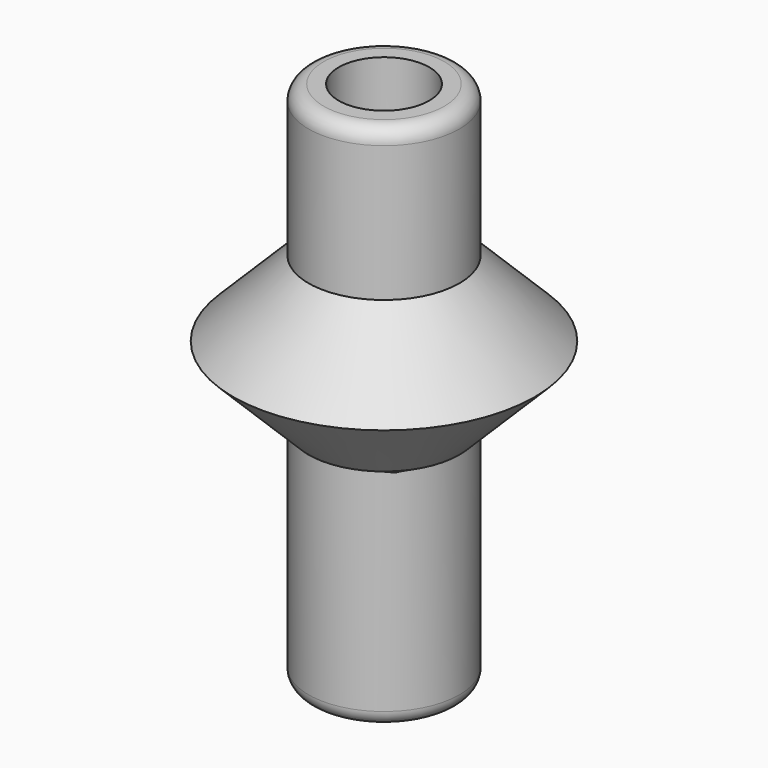
from build123d import *

# Parameters (mm, degrees)
F0_R         = 12.7
F1_DEPTH     = 38.1
F2_R         = 25.4
F2_R_2       = 12.7
F3_DEPTH     = 12.7
F4_R         = 2.54
F5_T1_DEPTH  = 10.7763073453
F5_T3_DEPTH  = 10.7763073453
F5_T9_DEPTH  = 23.4763073453
F5_S10_R     = 12.7
F5_T11_DEPTH = 14
F5_T15_DEPTH = 23.4763073453
F5_S16_R     = 12.7
F5_T17_DEPTH = 14
F5_T24_DEPTH = 23.4763073453
F5_S25_R     = 12.7
F5_T26_DEPTH = 14
F5_T30_DEPTH = 23.4763073453
F5_S31_R     = 12.7
F5_T32_DEPTH = 14
F5_T39_DEPTH = 23.4763073453
F5_S40_R     = 12.7
F5_T41_DEPTH = 14
F5_T45_DEPTH = 23.4763073453
F5_S46_R     = 12.7
F5_T47_DEPTH = 14
F5_T54_DEPTH = 23.4763073453
F5_S55_R     = 12.7
F5_T56_DEPTH = 14
F5_T60_DEPTH = 23.4763073453
F5_S61_R     = 12.7
F5_T62_DEPTH = 14
F8_R         = 12.7
F8_R_2       = 7.62
F9_DEPTH     = 25.4
F10_R        = 2.54
F11_DEPTH    = 25.4
F12_SIZE     = 12.69999
F13_R        = 2.54
F14_DEPTH    = 152.4


# Not quite as in the source:
# - a fillet or chamfer that OpenCascade refuses, or shapes differently, is made with other operations: its cross-section is extruded or revolved along the edge and cut away or added
# - a fillet or chamfer is up to 0.001 mm smaller than in the source, because OpenCascade refuses the exact size


with BuildPart() as f1:
    # F0 (on Top) → F1 (new body)
    with BuildSketch(Plane.XY):
        Circle(F0_R)
        with BuildLine():
            ThreePointArc((5.3881536726, 5.3881536726), (7.0399620377, 2.9160477546), (7.62, 0))
            ThreePointArc((7.62, 0), (7.0399620377, -2.9160477546), (5.3881536726, -5.3881536726))
            ThreePointArc((5.3881536726, -5.3881536726), (0, -7.62), (-5.3881536726, -5.3881536726))
            ThreePointArc((-5.3881536726, -5.3881536726), (-7.62, 0), (-5.3881536726, 5.3881536726))
            ThreePointArc((-5.3881536726, 5.3881536726), (0, 7.62), (5.3881536726, 5.3881536726))
        make_face(mode=Mode.SUBTRACT)
        with BuildLine():
            ThreePointArc((-5.3881536726, -5.3881536726), (0, -7.62), (5.3881536726, -5.3881536726))
            Line((5.3881536726, -5.3881536726), (-5.3881536726, -5.3881536726))
        make_face()
        with BuildLine():
            Line((-5.3881536726, -5.3881536726), (-5.3881536726, 5.3881536726))
            ThreePointArc((-5.3881536726, 5.3881536726), (-7.62, 0), (-5.3881536726, -5.3881536726))
        make_face()
        with BuildLine():
            ThreePointArc((5.3881536726, -5.3881536726), (7.0399620377, -2.9160477546), (7.62, 0))
            ThreePointArc((7.62, 0), (7.0399620377, 2.9160477546), (5.3881536726, 5.3881536726))
            Line((5.3881536726, 5.3881536726), (5.3881536726, -5.3881536726))
        make_face()
        with BuildLine():
            Line((-5.3881536726, 5.3881536726), (5.3881536726, 5.3881536726))
            ThreePointArc((5.3881536726, 5.3881536726), (0, 7.62), (-5.3881536726, 5.3881536726))
        make_face()
    extrude(amount=F1_DEPTH)

    # F4
    f4_edges = [f1.edges().sort_by_distance(p)[0] for p in [
        (-12.7, 0, 0),
    ]]
    fillet(f4_edges, radius=F4_R)

    # F5: fillet of radius 5.08 on 4 edges, made by hand

    # F5_s2 → F5_t1 (cut)
    with BuildSketch(Plane.XZ.offset(-5.3881536726)):
        with BuildLine():
            ThreePointArc((10.4681536726, 38.1), (6.8760512242, 36.6121024484), (5.3881536726, 33.02))
            Line((5.3881536726, 33.02), (5.3881536726, 38.1))
            Line((5.3881536726, 38.1), (10.4681536726, 38.1))
        make_face()
        with BuildLine():
            ThreePointArc((-10.4681536726, 38.1), (-6.8760512242, 36.6121024484), (-5.3881536726, 33.02))
            Line((-5.3881536726, 33.02), (-5.3881536726, 38.1))
            Line((-5.3881536726, 38.1), (-10.4681536726, 38.1))
        make_face()
    extrude(amount=F5_T1_DEPTH, mode=Mode.SUBTRACT)

    # F5_s4 → F5_t3 (cut)
    with BuildSketch(Plane.YZ.offset(-5.3881536726)):
        with BuildLine():
            ThreePointArc((-10.4681536726, 38.1), (-6.8760512242, 36.6121024484), (-5.3881536726, 33.02))
            Line((-5.3881536726, 33.02), (-5.3881536726, 38.1))
            Line((-5.3881536726, 38.1), (-10.4681536726, 38.1))
        make_face()
        with BuildLine():
            ThreePointArc((10.4681536726, 38.1), (6.8760512242, 36.6121024484), (5.3881536726, 33.02))
            Line((5.3881536726, 33.02), (5.3881536726, 38.1))
            Line((5.3881536726, 38.1), (10.4681536726, 38.1))
        make_face()
    extrude(amount=F5_T3_DEPTH, mode=Mode.SUBTRACT)


with BuildPart() as f3:
    # F2 (on face) → F3 (new body)
    with BuildSketch(Plane.XY.offset(38.1)):
        Circle(F2_R)
        Circle(F2_R_2, mode=Mode.SUBTRACT)
    extrude(amount=F3_DEPTH)

    # F6: F3 across face


with BuildPart() as f5_tool7:
    # F5_s8 → F5_t9 (new body)
    with BuildSketch(Plane.YZ.offset(-5.3881536726)):
        with BuildLine():
            ThreePointArc((10.4681536726, 38.1), (6.8760512242, 36.6121024484), (5.3881536726, 33.02))
            Line((5.3881536726, 33.02), (5.3881536726, 38.1))
            Line((5.3881536726, 38.1), (10.4681536726, 38.1))
        make_face()
    extrude(amount=F5_T9_DEPTH)

    # F5_s10 → F5_t11 (intersect, symmetric)
    with BuildSketch(Plane.XY.offset(35.6)):
        Circle(F5_S10_R)
    extrude(amount=F5_T11_DEPTH, both=True, mode=Mode.INTERSECT)

    split(bisect_by=Plane.YZ.offset(5.3881536726), keep=Keep.TOP)


with BuildPart() as f5_tool13:
    # F5_s14 → F5_t15 (new body)
    with BuildSketch(Plane.XZ.offset(-18.0881536726)):
        with BuildLine():
            ThreePointArc((10.4681536726, 38.1), (6.8760512242, 36.6121024484), (5.3881536726, 33.02))
            Line((5.3881536726, 33.02), (5.3881536726, 38.1))
            Line((5.3881536726, 38.1), (10.4681536726, 38.1))
        make_face()
    extrude(amount=F5_T15_DEPTH)

    # F5_s16 → F5_t17 (intersect, symmetric)
    with BuildSketch(Plane.XY.offset(35.6)):
        Circle(F5_S16_R)
    extrude(amount=F5_T17_DEPTH, both=True, mode=Mode.INTERSECT)

    split(bisect_by=Plane.XZ.offset(-5.3881536726), keep=Keep.BOTTOM)


with BuildPart() as f5_tool7_1:
    add(f5_tool7.part)

    # F5_t19: intersect F5_tool13
    add(f5_tool13.part, mode=Mode.INTERSECT)


with BuildPart() as f1_1:
    add(f1.part)

    # F5_t5: cut F5_tool7
    add(f5_tool7_1.part, mode=Mode.SUBTRACT)


with BuildPart() as f5_tool22:
    # F5_s23 → F5_t24 (new body)
    with BuildSketch(Plane.YZ.offset(18.0881536726)):
        with BuildLine():
            ThreePointArc((-10.4681536726, 38.1), (-6.8760512242, 36.6121024484), (-5.3881536726, 33.02))
            Line((-5.3881536726, 33.02), (-5.3881536726, 38.1))
            Line((-5.3881536726, 38.1), (-10.4681536726, 38.1))
        make_face()
    extrude(amount=-F5_T24_DEPTH)

    # F5_s25 → F5_t26 (intersect, symmetric)
    with BuildSketch(Plane.XY.offset(35.6)):
        Circle(F5_S25_R)
    extrude(amount=F5_T26_DEPTH, both=True, mode=Mode.INTERSECT)

    split(bisect_by=Plane.YZ.offset(5.3881536726), keep=Keep.TOP)


with BuildPart() as f5_tool28:
    # F5_s29 → F5_t30 (new body)
    with BuildSketch(Plane.XZ.offset(-5.3881536726)):
        with BuildLine():
            ThreePointArc((10.4681536726, 38.1), (6.8760512242, 36.6121024484), (5.3881536726, 33.02))
            Line((5.3881536726, 33.02), (5.3881536726, 38.1))
            Line((5.3881536726, 38.1), (10.4681536726, 38.1))
        make_face()
    extrude(amount=F5_T30_DEPTH)

    # F5_s31 → F5_t32 (intersect, symmetric)
    with BuildSketch(Plane.XY.offset(35.6)):
        Circle(F5_S31_R)
    extrude(amount=F5_T32_DEPTH, both=True, mode=Mode.INTERSECT)

    split(bisect_by=Plane.XZ.offset(5.3881536726), keep=Keep.TOP)


with BuildPart() as f5_tool22_1:
    add(f5_tool22.part)

    # F5_t34: intersect F5_tool28
    add(f5_tool28.part, mode=Mode.INTERSECT)


with BuildPart() as f1_2:
    add(f1_1.part)

    # F5_t20: cut F5_tool22
    add(f5_tool22_1.part, mode=Mode.SUBTRACT)


with BuildPart() as f5_tool37:
    # F5_s38 → F5_t39 (new body)
    with BuildSketch(Plane.YZ.offset(5.3881536726)):
        with BuildLine():
            ThreePointArc((-10.4681536726, 38.1), (-6.8760512242, 36.6121024484), (-5.3881536726, 33.02))
            Line((-5.3881536726, 33.02), (-5.3881536726, 38.1))
            Line((-5.3881536726, 38.1), (-10.4681536726, 38.1))
        make_face()
    extrude(amount=-F5_T39_DEPTH)

    # F5_s40 → F5_t41 (intersect, symmetric)
    with BuildSketch(Plane.XY.offset(35.6)):
        Circle(F5_S40_R)
    extrude(amount=F5_T41_DEPTH, both=True, mode=Mode.INTERSECT)

    split(bisect_by=Plane.YZ.offset(-5.3881536726), keep=Keep.BOTTOM)


with BuildPart() as f5_tool43:
    # F5_s44 → F5_t45 (new body)
    with BuildSketch(Plane.XZ.offset(18.0881536726)):
        with BuildLine():
            ThreePointArc((-10.4681536726, 38.1), (-6.8760512242, 36.6121024484), (-5.3881536726, 33.02))
            Line((-5.3881536726, 33.02), (-5.3881536726, 38.1))
            Line((-5.3881536726, 38.1), (-10.4681536726, 38.1))
        make_face()
    extrude(amount=-F5_T45_DEPTH)

    # F5_s46 → F5_t47 (intersect, symmetric)
    with BuildSketch(Plane.XY.offset(35.6)):
        Circle(F5_S46_R)
    extrude(amount=F5_T47_DEPTH, both=True, mode=Mode.INTERSECT)

    split(bisect_by=Plane.XZ.offset(5.3881536726), keep=Keep.TOP)


with BuildPart() as f5_tool37_1:
    add(f5_tool37.part)

    # F5_t49: intersect F5_tool43
    add(f5_tool43.part, mode=Mode.INTERSECT)


with BuildPart() as f1_3:
    add(f1_2.part)

    # F5_t35: cut F5_tool37
    add(f5_tool37_1.part, mode=Mode.SUBTRACT)


with BuildPart() as f5_tool52:
    # F5_s53 → F5_t54 (new body)
    with BuildSketch(Plane.XZ.offset(5.3881536726)):
        with BuildLine():
            ThreePointArc((-10.4681536726, 38.1), (-6.8760512242, 36.6121024484), (-5.3881536726, 33.02))
            Line((-5.3881536726, 33.02), (-5.3881536726, 38.1))
            Line((-5.3881536726, 38.1), (-10.4681536726, 38.1))
        make_face()
    extrude(amount=-F5_T54_DEPTH)

    # F5_s55 → F5_t56 (intersect, symmetric)
    with BuildSketch(Plane.XY.offset(35.6)):
        Circle(F5_S55_R)
    extrude(amount=F5_T56_DEPTH, both=True, mode=Mode.INTERSECT)

    split(bisect_by=Plane.XZ.offset(-5.3881536726), keep=Keep.BOTTOM)


with BuildPart() as f5_tool58:
    # F5_s59 → F5_t60 (new body)
    with BuildSketch(Plane.YZ.offset(-18.0881536726)):
        with BuildLine():
            ThreePointArc((10.4681536726, 38.1), (6.8760512242, 36.6121024484), (5.3881536726, 33.02))
            Line((5.3881536726, 33.02), (5.3881536726, 38.1))
            Line((5.3881536726, 38.1), (10.4681536726, 38.1))
        make_face()
    extrude(amount=F5_T60_DEPTH)

    # F5_s61 → F5_t62 (intersect, symmetric)
    with BuildSketch(Plane.XY.offset(35.6)):
        Circle(F5_S61_R)
    extrude(amount=F5_T62_DEPTH, both=True, mode=Mode.INTERSECT)

    split(bisect_by=Plane.YZ.offset(-5.3881536726), keep=Keep.BOTTOM)


with BuildPart() as f5_tool52_1:
    add(f5_tool52.part)

    # F5_t64: intersect F5_tool58
    add(f5_tool58.part, mode=Mode.INTERSECT)


with BuildPart() as f1_4:
    add(f1_3.part)

    # F5_t50: cut F5_tool52
    add(f5_tool52_1.part, mode=Mode.SUBTRACT)


with BuildPart() as f3_1:
    add(f3.part)
    add(f3.part.mirror(Plane.XY.offset(50.8)))

    # F12 (size 12.7 in the source; OpenCascade refuses exactly that, so slightly less here)
    f12_edges = [f3_1.edges().sort_by_distance(p)[0] for p in [
        (-25.4, 0, 38.1),
        (-25.4, 0, 63.5),
    ]]
    chamfer(f12_edges, length=F12_SIZE)

    # F13 (on face) → F14 (cut)
    with BuildSketch(Plane.XY.offset(88.9)):
        with Locations((0, 17.78)):
            Circle(F13_R)
    extrude(amount=-F14_DEPTH, mode=Mode.SUBTRACT)


with BuildPart() as f9:
    # F8 (on offset) → F9 (new body)
    with BuildSketch(Plane.XY.offset(63.5)):
        Circle(F8_R)
        Circle(F8_R_2, mode=Mode.SUBTRACT)
    extrude(amount=F9_DEPTH)

    # F10
    f10_edges = [f9.edges().sort_by_distance(p)[0] for p in [
        (-12.7, 0, 88.9),
    ]]
    fillet(f10_edges, radius=F10_R)

    # F8 (on offset) → F11 (join)
    with BuildSketch(Plane.XY.offset(63.5)):
        Circle(F8_R)
        Circle(F8_R_2, mode=Mode.SUBTRACT)
    extrude(amount=-F11_DEPTH)


solid = Compound([f1_4.part, f3_1.part, f9.part])
